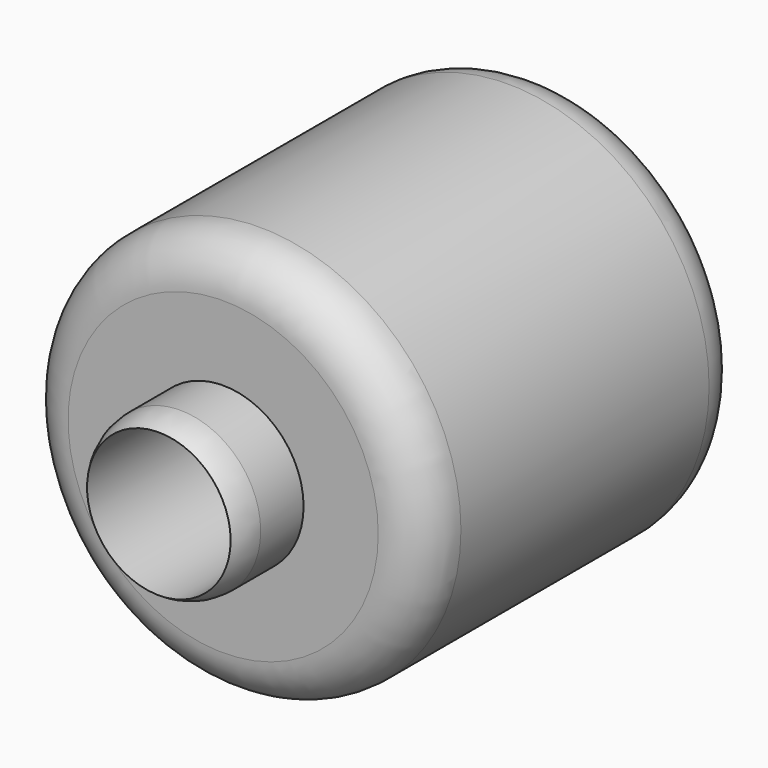
from build123d import *

# Parameters (mm, degrees)
F0_R     = 8.89
F0_R_2   = 7.9375
F1_DEPTH = 53.34
F0_R_3   = 22.225
F2_DEPTH = 44.45
F3_R     = 5.08
F4_R     = 5.08


# Not quite as in the source:
# - a fillet or chamfer that OpenCascade refuses, or shapes differently, is made with other operations: its cross-section is extruded or revolved along the edge and cut away or added


with BuildPart() as f1:
    # F0 (on Front) → F1 (new body)
    with BuildSketch(Plane.XZ):
        Circle(F0_R)
        Circle(F0_R_2, mode=Mode.SUBTRACT)
    extrude(amount=F1_DEPTH)

    # F0 (on Front) → F2 (join)
    with BuildSketch(Plane.XZ):
        Circle(F0_R_3)
        Circle(F0_R, mode=Mode.SUBTRACT)
    extrude(amount=F2_DEPTH)

    # F3
    f3_edges = [f1.edges().sort_by_distance(p)[0] for p in [
        (-22.225, -44.45, 0),
    ]]
    fillet(f3_edges, radius=F3_R)

    # F4
    f4_edges = [f1.edges().sort_by_distance(p)[0] for p in [
        (-22.225, 0, 0),
    ]]
    fillet(f4_edges, radius=F4_R)

    # F5: fillet of radius 5.08 on 1 edges, made by hand

    # F5_s1 → F5_t2 (revolve, cut)
    with BuildSketch(Plane.XY):
        with BuildLine():
            ThreePointArc((8.89, -50.3785571506), (8.6460159222, -51.9339831373), (7.9375, -53.34))
            Line((7.9375, -53.34), (8.89, -53.34))
            Line((8.89, -53.34), (8.89, -50.3785571506))
        make_face()
    revolve(axis=Axis((0, -53.34, 0), (0, -1, 0)), mode=Mode.SUBTRACT)


solid = f1.part
